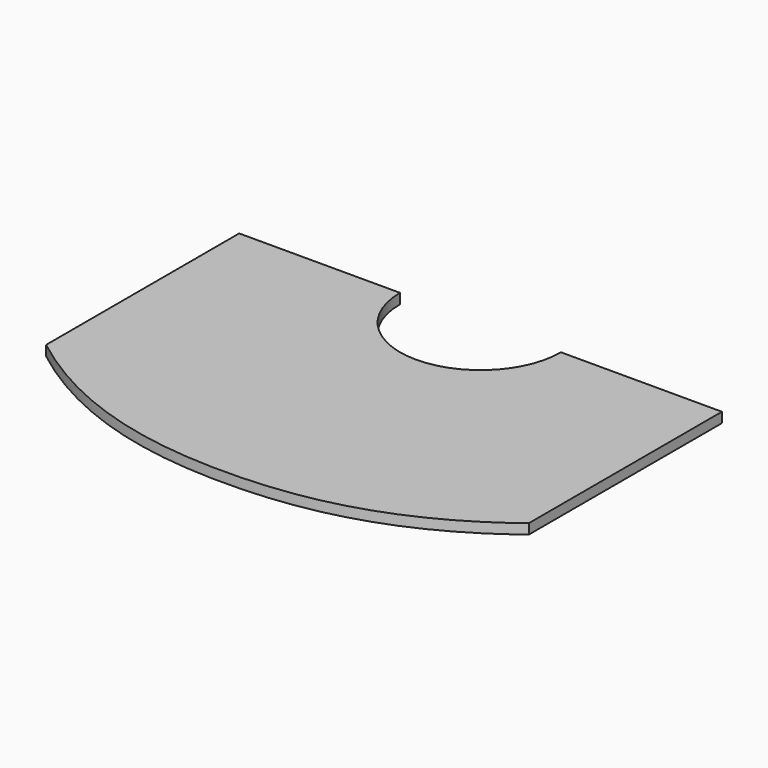
from build123d import *

# Parameters (mm, degrees)
F1_DEPTH = 3.175


# Not quite as in the source:
# - a length typed as a fraction of an inch, garbled in the dataset ("3 / 203.2 mm" for 3/8 in), is restored


with BuildPart() as f1:
    # F0 (on Top) → F1 (new body)
    with BuildSketch(Plane.XY):
        with BuildLine():
            Line((-67.493813857, 42.5679214677), (-92.893813857, 42.5679214677))
            Line((-92.893813857, 42.5679214677), (-92.893813857, -33.6320785323))
            add(Edge.make_bspline(
                [(-92.893813857, -33.6320785323), (-67.493813857, -53.2479426065), (-16.693813857, -64.816214458), (34.106186143, -53.2479426065), (59.506186143, -33.6320785323)],
                knots=[0, 0, 0, 0, 0.5, 1, 1, 1, 1], degree=3))
            Line((59.506186143, -33.6320785323), (59.506186143, 42.5679214677))
            Line((59.506186143, 42.5679214677), (34.106186143, 42.5679214677))
            Line((34.106186143, 42.5679214677), (8.706186143, 42.5679214677))
            ThreePointArc((8.706186143, 42.5679214677), (1.2666983851, 24.6074092256), (-16.693813857, 17.1679214677))
            ThreePointArc((-16.693813857, 17.1679214677), (-34.6543260992, 24.6074092256), (-42.093813857, 42.5679214677))
            Line((-42.093813857, 42.5679214677), (-67.493813857, 42.5679214677))
        make_face()
    extrude(amount=F1_DEPTH)


solid = f1.part
